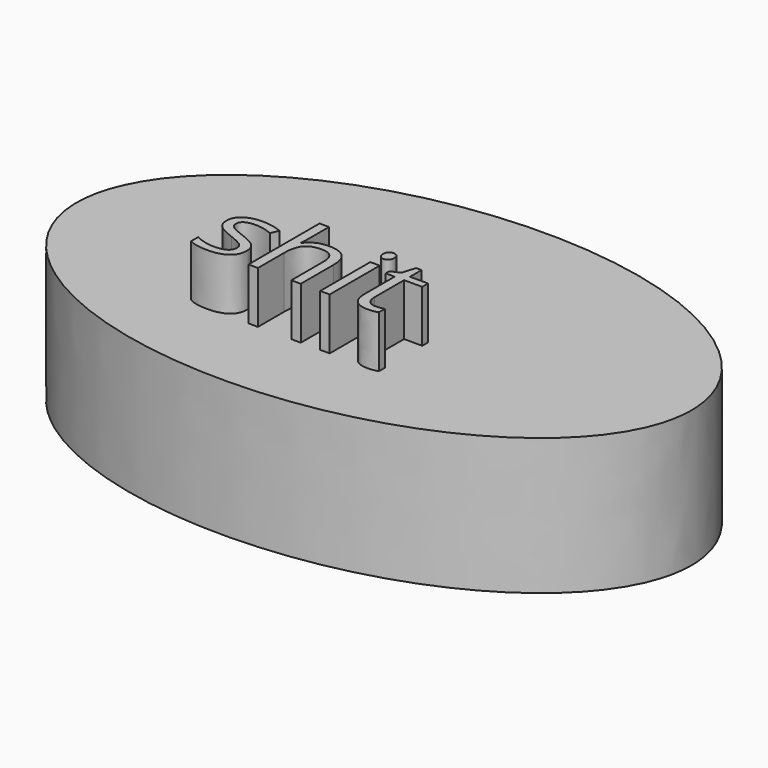
from build123d import *

# Parameters (mm, degrees)
F1_DEPTH     = 25.4
F2_TEXT_SIZE = 21.7425158351
F3_DEPTH     = 9.652


# Not quite as in the source:
# - Text() gives the source's letters only with a copy of the font that has no kerning and outlines rounded to 1/6400 em; it was checked with that copy


with BuildPart() as f1:
    # F0 (on Top) → F1 (new body)
    with BuildSketch(Plane.XY):
        with BuildLine():
            add(Edge.make_bspline(
                [(37.3952500522, -3.9684735239), (33.6681696471, 52.2482989372), (-47.3483754845, 18.6450981077), (-128.3649206161, -14.9581027217), (-43.6212950794, -37.5716743533), (41.1223304573, -60.1852459849), (37.3952500522, -3.9684735239)],
                knots=[0, 0, 0, 2.0943951024, 2.0943951024, 4.1887902048, 4.1887902048, 6.2831853072, 6.2831853072, 6.2831853072], degree=2, weights=[1, 0.5, 1, 0.5, 1, 0.5, 1]))
        make_face()
    extrude(amount=F1_DEPTH)

    # F2 (on face) → F3 (join)
    with BuildSketch(Plane.XY.offset(25.4)):
        with Locations((-42.1428605914, -24.0890979767)):
            Text('shit', F2_TEXT_SIZE, font='Open Sans', text_align=(TextAlign.LEFT, TextAlign.BOTTOM))
    extrude(amount=F3_DEPTH)


solid = f1.part
